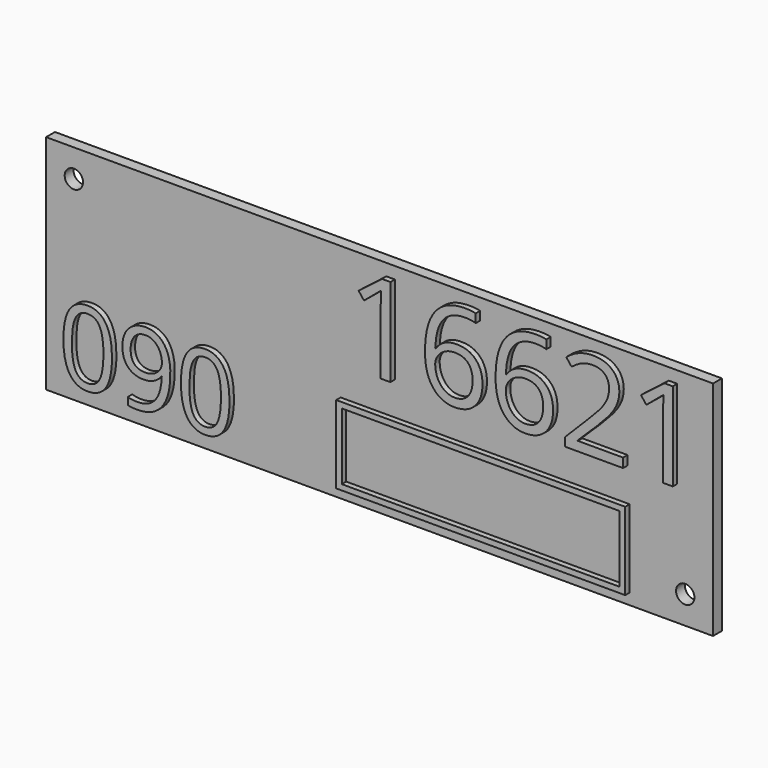
from build123d import *

# Parameters (mm, degrees)
F0_W         = 120
F0_H         = 40
F1_DEPTH     = 2
F3_D         = 3.3
F4_TEXT_SIZE = 22.2157940411
F5_DEPTH     = 1
F6_TEXT_SIZE = 18.4937691891
F7_DEPTH     = 1
F8_W         = 52
F8_H         = 14
F8_W_2       = 49.99999962
F8_H_2       = 11.99999962
F9_DEPTH     = 1


# Not quite as in the source:
# - Text() gives the source's letters only with a copy of the font that has no kerning and outlines rounded to 1/6400 em; it was checked with that copy


with BuildPart() as f1:
    # F0 (on Front) → F1 (new body)
    with BuildSketch(Plane.XZ):
        Rectangle(F0_W, F0_H)
    extrude(amount=F1_DEPTH)

    # F3 (through all)
    with Locations(Plane.XZ.offset(2)):
        with Locations((-55, 15), (55, -15)):
            Hole(F3_D / 2)

    # F4 (on face) → F5 (join)
    with BuildSketch(Plane.XZ.offset(2)):
        with Locations((-5, 2)):
            Text('16621', F4_TEXT_SIZE, font='Open Sans', text_align=(TextAlign.LEFT, TextAlign.BOTTOM))
    extrude(amount=F5_DEPTH)

    # F6 (on face) → F7 (join)
    with BuildSketch(Plane.XZ.offset(2)):
        with Locations((-57, -17)):
            Text('090', F6_TEXT_SIZE, font='Open Sans', text_align=(TextAlign.LEFT, TextAlign.BOTTOM))
    extrude(amount=F7_DEPTH)

    # F8 (on face) → F9 (join)
    with BuildSketch(Plane.XZ.offset(2)):
        with Locations((19, -11)):
            Rectangle(F8_W, F8_H)
        with Locations((19, -11)):
            Rectangle(F8_W_2, F8_H_2, mode=Mode.SUBTRACT)
    extrude(amount=F9_DEPTH)


solid = f1.part
